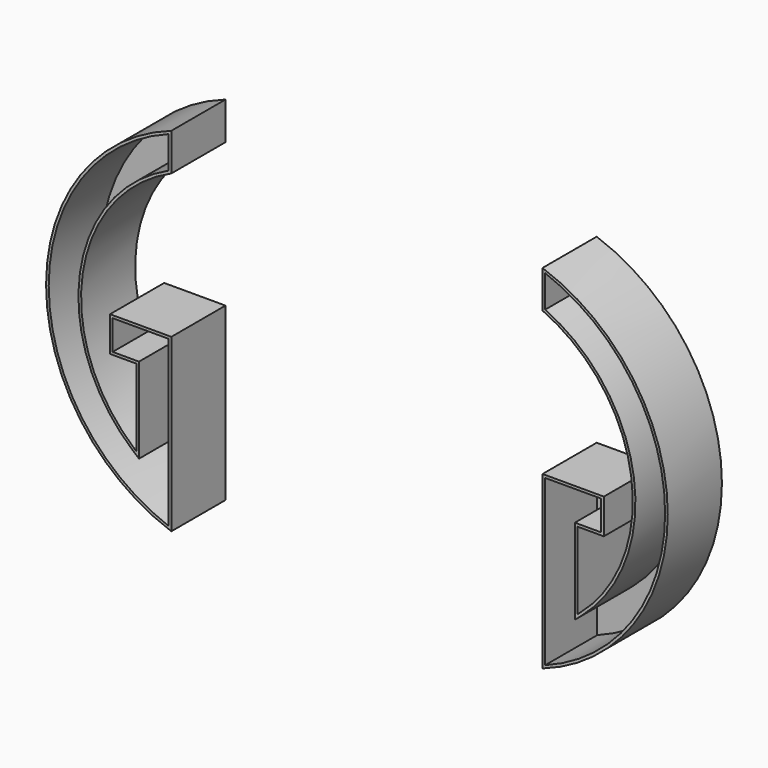
from build123d import *

# Parameters (mm, degrees)
F1_DEPTH = 18
F2_T     = -0.7


# Not quite as in the source:
# - ends of sketch curves that miss each other by under 0.0002 mm in the source are joined


with BuildPart() as f1:
    # F0 (on Front) → F1 (new body)
    with BuildSketch(Plane.XZ):
        with BuildLine():
            Line((-49.350248, 36.881888), (-49.350248, 46.873415))
            ThreePointArc((-49.350248, 46.873415), (-82.649751, -0.006585), (-49.350248, -46.886585))
            Line((-49.350248, -46.886585), (-49.350248, -1.356565))
            Line((-49.350248, -1.356565), (-65.650005, -1.356565))
            Line((-65.650005, -1.356565), (-65.650005, -10.656426))
            Line((-65.650005, -10.656426), (-58.65011, -10.656426))
            Line((-58.65011, -10.656426), (-58.65011, -31.163423))
            Line((-58.65011, -31.163423), (-59.227601, -30.669473))
            ThreePointArc((-59.227601, -30.669473), (-72.925346, 5.831223), (-49.350248, 36.881888))
        make_face()
        with BuildLine():
            ThreePointArc((-50.60023, -45.092496), (-81.39977, -0.006585), (-50.60023, 45.079326))
            Line((-50.60023, 45.079326), (-50.60023, 37.686354))
            ThreePointArc((-50.60023, 37.686354), (-74.219281, 5.607663), (-60.040089, -31.619376))
            Line((-60.040089, -31.619376), (-57.400128, -33.877433))
            Line((-57.400128, -33.877433), (-57.400128, -9.406445))
            Line((-57.400128, -9.406445), (-64.400024, -9.406445))
            Line((-64.400024, -9.406445), (-64.400024, -2.606546))
            Line((-64.400024, -2.606546), (-50.60023, -2.606546))
            Line((-50.60023, -2.606546), (-50.60023, -45.092496))
        make_face(mode=Mode.SUBTRACT)
        with BuildLine():
            Line((-50.60023, 37.686354), (-50.60023, 45.079326))
            ThreePointArc((-50.60023, 45.079326), (-81.39977, -0.006585), (-50.60023, -45.092496))
            Line((-50.60023, -45.092496), (-50.60023, -2.606546))
            Line((-50.60023, -2.606546), (-64.400024, -2.606546))
            Line((-64.400024, -2.606546), (-64.400024, -9.406445))
            Line((-64.400024, -9.406445), (-57.400128, -9.406445))
            Line((-57.400128, -9.406445), (-57.400128, -33.877433))
            Line((-57.400128, -33.877433), (-60.040089, -31.619376))
            ThreePointArc((-60.040089, -31.619376), (-74.219281, 5.607663), (-50.60023, 37.686354))
        make_face()
        with BuildLine():
            ThreePointArc((-50.950225, -44.577211), (-81.049775, -0.006585), (-50.950225, 44.564041))
            Line((-50.950225, 44.564041), (-50.950225, 37.908545))
            ThreePointArc((-50.950225, 37.908545), (-74.580984, 5.544337), (-60.267586, -31.885349))
            Line((-60.267586, -31.885349), (-57.050134, -34.637356))
            Line((-57.050134, -34.637356), (-57.050134, -9.05645))
            Line((-57.050134, -9.05645), (-64.050029, -9.05645))
            Line((-64.050029, -9.05645), (-64.050029, -2.956541))
            Line((-64.050029, -2.956541), (-50.950225, -2.956541))
            Line((-50.950225, -2.956541), (-50.950225, -44.577211))
        make_face(mode=Mode.SUBTRACT)
        with BuildLine():
            Line((-50.950225, 37.908545), (-50.950225, 44.564041))
            ThreePointArc((-50.950225, 44.564041), (-81.049775, -0.006585), (-50.950225, -44.577211))
            Line((-50.950225, -44.577211), (-50.950225, -2.956541))
            Line((-50.950225, -2.956541), (-64.050029, -2.956541))
            Line((-64.050029, -2.956541), (-64.050029, -9.05645))
            Line((-64.050029, -9.05645), (-57.050134, -9.05645))
            Line((-57.050134, -9.05645), (-57.050134, -34.637356))
            Line((-57.050134, -34.637356), (-60.267585, -31.885349))
            ThreePointArc((-60.267585, -31.885349), (-74.580984, 5.544337), (-50.950225, 37.908545))
        make_face()
    extrude(amount=F1_DEPTH)

    # F2
    f2_openings = [f1.faces().sort_by_distance(p)[0] for p in [
        (-64.64766, -18, -4.27446),
    ]]
    offset(amount=F2_T, openings=f2_openings, kind=Kind.INTERSECTION)


with BuildPart() as f3_1:
    # F3: instance of F1
    add(f1.part.mirror(Plane.YZ))


solid = Compound([f1.part, f3_1.part])
